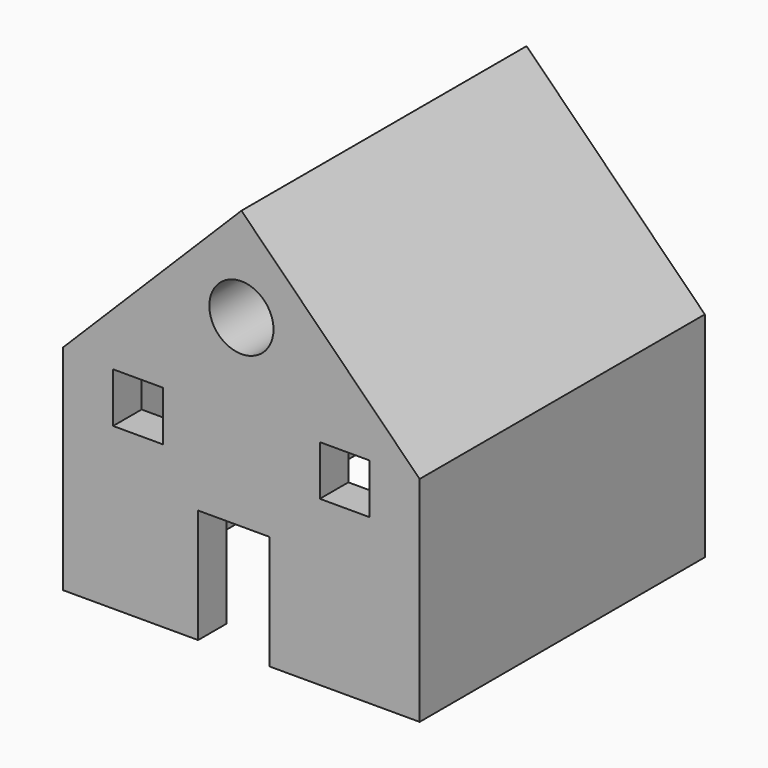
from build123d import *

# Parameters (mm, degrees)
F0_W     = 50
F0_H     = 50
F0_W_2   = 40
F0_H_2   = 40
F1_DEPTH = 30
F2_W     = 50
F2_H     = 50
F3_DEPTH = 25
F4_SIZE  = 24.99999
F5_W     = 10
F5_H     = 16
F6_DEPTH = 5
F5_W_2   = 7
F5_H_2   = 7
F7_DEPTH = 50.001
F5_R     = 4.5
F8_DEPTH = 50.001


# Not quite as in the source:
# - a fillet or chamfer is up to 0.001 mm smaller than in the source, because OpenCascade refuses the exact size


with BuildPart() as f1:
    # F0 (on Top) → F1 (new body)
    with BuildSketch(Plane.XY):
        with Locations((25, 25)):
            Rectangle(F0_W, F0_H)
        with Locations((25, 25)):
            Rectangle(F0_W_2, F0_H_2, mode=Mode.SUBTRACT)
    extrude(amount=F1_DEPTH)

    # F2 (on face) → F3 (join)
    with BuildSketch(Plane.XY.offset(30)):
        with Locations((25, 25)):
            Rectangle(F2_W, F2_H)
    extrude(amount=F3_DEPTH)

    # F4 (size 25 in the source; OpenCascade refuses exactly that, so slightly less here)
    f4_edges = [f1.edges().sort_by_distance(p)[0] for p in [
        (0, 25, 55),
        (50, 25, 55),
    ]]
    chamfer(f4_edges, length=F4_SIZE)

    # F5 (on face) → F6 (cut)
    with BuildSketch(Plane.XZ):
        with Locations((23.930438906, 8)):
            Rectangle(F5_W, F5_H)
    extrude(amount=-F6_DEPTH, mode=Mode.SUBTRACT)

    # F5 (on face) → F7 (cut, through all)
    with BuildSketch(Plane.XZ):
        with Locations((10.5, 26.0614674687)):
            Rectangle(F5_W_2, F5_H_2)
        with Locations((39.5, 26.5)):
            Rectangle(F5_W_2, F5_H_2)
    extrude(amount=-F7_DEPTH, mode=Mode.SUBTRACT)

    # F5 (on face) → F8 (cut, through all)
    with BuildSketch(Plane.XZ):
        with Locations((25, 41.7942066526)):
            Circle(F5_R)
    extrude(amount=-F8_DEPTH, mode=Mode.SUBTRACT)


solid = f1.part
